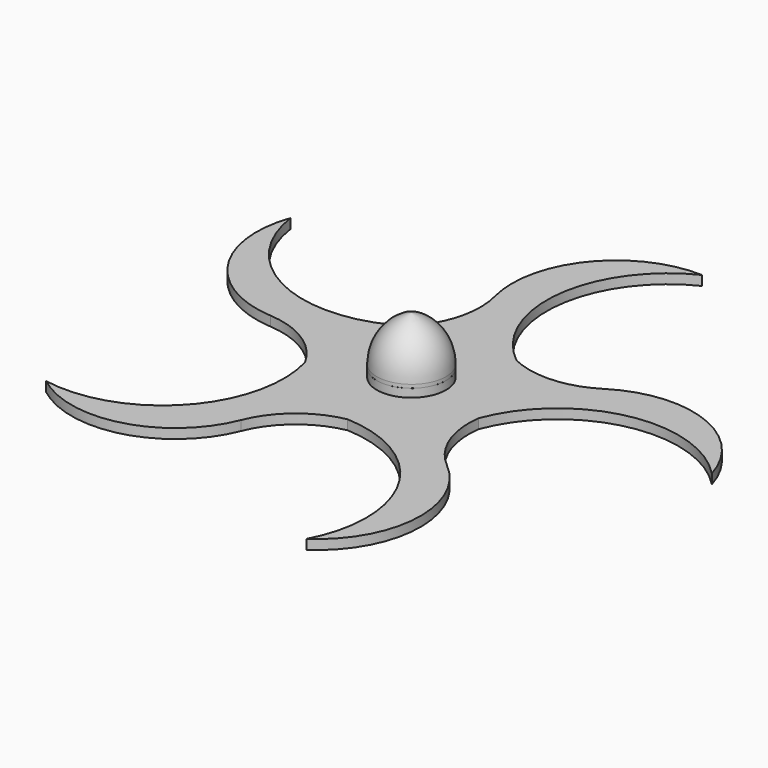
from build123d import *

# Parameters (mm, degrees)
F0_R     = 2.495
F1_DEPTH = 2.8
F3_DEPTH = 2.4
F5_DEPTH = 1
F6_W     = 7.505
F6_H     = 1


with BuildPart() as f1:
    # F0 (on Top) → F1 (new body)
    with BuildSketch(Plane.XY):
        with BuildLine():
            ThreePointArc((-22.7858082993, 10.2862500528), (-20.3407682899, 14.5345500576), (-17.1137876985, 18.2241123408))
            ThreePointArc((-17.1137876985, 18.2241123408), (-16.5666860585, 18.7537908739), (-16.0359703203, 19.2998864317))
            ThreePointArc((-16.0359703203, 19.2998864317), (-49.6996912533, 16.6900208036), (-69.9041814161, 43.7424898759))
            ThreePointArc((-69.9041814161, 43.7424898759), (-66.7598038962, 17.1440537541), (-43.6190942577, 3.6580806138))
            ThreePointArc((-43.6190942577, 3.6580806138), (-32.5771806136, 5.0068500705), (-22.7858082993, 10.2862500528))
        make_face()
        with BuildLine():
            ThreePointArc((-23.7810968086, -7.7109943963), (-24.9618581995, 1.3804474739), (-22.7858082993, 10.2862500528))
            ThreePointArc((-22.7858082993, 10.2862500528), (-32.5771806136, 5.0068500705), (-43.6190942577, 3.6580806138))
            ThreePointArc((-43.6190942577, 3.6580806138), (-31.8033376807, -0.2078903454), (-23.3106701049, -9.2871211714))
            ThreePointArc((-23.3106701049, -9.2871211714), (-23.5366233714, -8.4962939253), (-23.7810968086, -7.7109943963))
        make_face()
        with BuildLine():
            ThreePointArc((-14.6823545264, 20.2343387725), (-6.4007548293, 24.1667196288), (2.7416031459, 24.8492175368))
            ThreePointArc((2.7416031459, 24.8492175368), (-5.3051050528, 32.5299416652), (-10, 42.6146329052))
            ThreePointArc((-10, 42.6146329052), (-10.0254872889, 30.1825298915), (-16.0359703203, 19.2998864317))
            ThreePointArc((-16.0359703203, 19.2998864317), (-15.353672314, 19.7591598168), (-14.6823545264, 20.2343387725))
        make_face()
        with BuildLine():
            ThreePointArc((-17.1137876985, 18.2241123408), (-15.9298122297, 19.2676174533), (-14.6823545264, 20.2343387725))
            ThreePointArc((-14.6823545264, 20.2343387725), (-15.353672314, 19.7591598168), (-16.0359703203, 19.2998864317))
            ThreePointArc((-16.0359703203, 19.2998864317), (-16.5666860585, 18.7537908739), (-17.1137876985, 18.2241123408))
        make_face()
        with BuildLine():
            ThreePointArc((24.5572095563, -4.684384571), (24.8890562186, -2.3526326842), (25, 0))
            ThreePointArc((25, 0), (24.8697135657, 2.5489894392), (24.4802122271, 5.0714109788))
            ThreePointArc((24.4802122271, 5.0714109788), (21.0059741613, 13.5554066532), (14.7069026764, 20.2165034976))
            ThreePointArc((14.7069026764, 20.2165034976), (13.4020104362, 21.1041729586), (12.0437095584, 21.9077397299))
            ThreePointArc((12.0437095584, 21.9077397299), (7.5375354635, 23.8366432019), (2.7416031459, 24.8492175368))
            ThreePointArc((2.7416031459, 24.8492175368), (-6.4007548293, 24.1667196288), (-14.6823545264, 20.2343387725))
            ThreePointArc((-14.6823545264, 20.2343387725), (-15.9298122297, 19.2676174533), (-17.1137876985, 18.2241123408))
            ThreePointArc((-17.1137876985, 18.2241123408), (-20.3407682899, 14.5345500576), (-22.7858082993, 10.2862500528))
            ThreePointArc((-22.7858082993, 10.2862500528), (-24.9618581995, 1.3804474739), (-23.7810968086, -7.7109943963))
            ThreePointArc((-23.7810968086, -7.7109943963), (-23.2471758286, -9.1961304903), (-22.6206120324, -10.6446188885))
            ThreePointArc((-22.6206120324, -10.6446188885), (-20.1088216239, -14.8537972551), (-16.824007136, -18.4919653874))
            ThreePointArc((-16.824007136, -18.4919653874), (-9.0265219603, -23.3135561702), (-0.015171591, -24.9999953965))
            ThreePointArc((-0.015171591, -24.9999953965), (1.5622674252, -24.9511386612), (3.1334806162, -24.8028486112))
            ThreePointArc((3.1334806162, -24.8028486112), (7.9128330526, -23.7147016233), (12.3880000622, -21.714913181))
            ThreePointArc((12.3880000622, -21.714913181), (19.3831608278, -15.7890175857), (23.7717202497, -7.7398524773))
            ThreePointArc((23.7717202497, -7.7398524773), (24.2127101969, -6.2245212604), (24.5572095563, -4.684384571))
        make_face()
        Circle(F0_R, mode=Mode.SUBTRACT)
        with BuildLine():
            ThreePointArc((2.7416031459, 24.8492175368), (7.5375354635, 23.8366432019), (12.0437095584, 21.9077397299))
            ThreePointArc((12.0437095584, 21.9077397299), (12.7165274833, 21.5510948184), (13.3998954043, 21.2151069652))
            ThreePointArc((13.3998954043, 21.2151069652), (0.5151038299, 52.4247152891), (20, 80))
            ThreePointArc((20, 80), (-4.3249499065, 68.7901504845), (-10, 42.6146329052))
            ThreePointArc((-10, 42.6146329052), (-5.3051050528, 32.5299416652), (2.7416031459, 24.8492175368))
        make_face()
        with BuildLine():
            ThreePointArc((14.7069026764, 20.2165034976), (21.0059741613, 13.5554066532), (24.4802122271, 5.0714109788))
            ThreePointArc((24.4802122271, 5.0714109788), (29.2984453771, 15.0977595306), (37.4387543702, 22.6792109397))
            ThreePointArc((37.4387543702, 22.6792109397), (25.6072457824, 18.8617196848), (13.3998954043, 21.2151069652))
            ThreePointArc((13.3998954043, 21.2151069652), (14.0475320292, 20.7081262812), (14.7069026764, 20.2165034976))
        make_face()
        with BuildLine():
            ThreePointArc((24.4802122271, 5.0714109788), (24.8697135657, 2.5489894392), (25, 0))
            ThreePointArc((25, 0), (24.8890562186, -2.3526326842), (24.5572095563, -4.684384571))
            ThreePointArc((24.5572095563, -4.684384571), (24.4259322621, -5.4344817814), (24.3175611259, -6.1882292523))
            ThreePointArc((24.3175611259, -6.1882292523), (50.0180429279, 15.7102350956), (82.2648611911, 5.7002292241))
            ThreePointArc((82.2648611911, 5.7002292241), (64.0868378543, 25.3705973366), (37.4387543702, 22.6792109397))
            ThreePointArc((37.4387543702, 22.6792109397), (29.2984453771, 15.0977595306), (24.4802122271, 5.0714109788))
        make_face()
        with BuildLine():
            ThreePointArc((24.3175611259, -6.1882292523), (24.0355245661, -6.9608339317), (23.7717202497, -7.7398524773))
            ThreePointArc((23.7717202497, -7.7398524773), (19.3831608278, -15.7890175857), (12.3880000622, -21.714913181))
            ThreePointArc((12.3880000622, -21.714913181), (23.4125401133, -23.1990131213), (33.1384226973, -28.5981097064))
            ThreePointArc((33.1384226973, -28.5981097064), (25.8516355407, -18.52534604), (24.3175611259, -6.1882292523))
        make_face()
        with BuildLine():
            ThreePointArc((33.1384226973, -28.5981097064), (23.4125401133, -23.1990131213), (12.3880000622, -21.714913181))
            ThreePointArc((12.3880000622, -21.714913181), (7.9128330526, -23.7147016233), (3.1334806162, -24.8028486112))
            ThreePointArc((3.1334806162, -24.8028486112), (2.3795288615, -24.9097892705), (1.629183895, -25.0396429732))
            ThreePointArc((1.629183895, -25.0396429732), (30.3977467503, -42.7152560287), (30.8424802959, -76.4770645958))
            ThreePointArc((30.8424802959, -76.4770645958), (43.932793932, -53.1102590157), (33.1384226973, -28.5981097064))
        make_face()
        with BuildLine():
            ThreePointArc((1.629183895, -25.0396429732), (0.8072390901, -25.0101582411), (-0.015171591, -24.9999953965))
            ThreePointArc((-0.015171591, -24.9999953965), (-9.0265219603, -23.3135561702), (-16.824007136, -18.4919653874))
            ThreePointArc((-16.824007136, -18.4919653874), (-14.8286998241, -29.435538145), (-16.9580828098, -40.3538147522))
            ThreePointArc((-16.9580828098, -40.3538147522), (-9.6300563535, -30.3110131909), (1.629183895, -25.0396429732))
        make_face()
        with BuildLine():
            ThreePointArc((-16.9580828098, -40.3538147522), (-14.8286998241, -29.435538145), (-16.824007136, -18.4919653874))
            ThreePointArc((-16.824007136, -18.4919653874), (-20.1088216239, -14.8537972551), (-22.6206120324, -10.6446188885))
            ThreePointArc((-22.6206120324, -10.6446188885), (-22.9553025485, -9.9606146404), (-23.3106701049, -9.2871211714))
            ThreePointArc((-23.3106701049, -9.2871211714), (-31.2312022548, -42.1097151595), (-63.2031600709, -52.9656545041))
            ThreePointArc((-63.2031600709, -52.9656545041), (-36.9348779836, -58.1945425595), (-16.9580828098, -40.3538147522))
        make_face()
        with BuildLine():
            ThreePointArc((-23.3106701049, -9.2871211714), (-22.9553025485, -9.9606146404), (-22.6206120324, -10.6446188885))
            ThreePointArc((-22.6206120324, -10.6446188885), (-23.2471758286, -9.1961304903), (-23.7810968086, -7.7109943963))
            ThreePointArc((-23.7810968086, -7.7109943963), (-23.5366233714, -8.4962939253), (-23.3106701049, -9.2871211714))
        make_face()
        with BuildLine():
            ThreePointArc((1.629183895, -25.0396429732), (2.3795288615, -24.9097892705), (3.1334806162, -24.8028486112))
            ThreePointArc((3.1334806162, -24.8028486112), (1.5622674252, -24.9511386612), (-0.015171591, -24.9999953965))
            ThreePointArc((-0.015171591, -24.9999953965), (0.8072390901, -25.0101582411), (1.629183895, -25.0396429732))
        make_face()
        with BuildLine():
            ThreePointArc((24.3175611259, -6.1882292523), (24.4259322621, -5.4344817814), (24.5572095563, -4.684384571))
            ThreePointArc((24.5572095563, -4.684384571), (24.2127101969, -6.2245212604), (23.7717202497, -7.7398524773))
            ThreePointArc((23.7717202497, -7.7398524773), (24.0355245661, -6.9608339317), (24.3175611259, -6.1882292523))
        make_face()
        with BuildLine():
            ThreePointArc((12.0437095584, 21.9077397299), (13.4020104362, 21.1041729586), (14.7069026764, 20.2165034976))
            ThreePointArc((14.7069026764, 20.2165034976), (14.0475320292, 20.7081262812), (13.3998954043, 21.2151069652))
            ThreePointArc((13.3998954043, 21.2151069652), (12.7165274833, 21.5510948184), (12.0437095584, 21.9077397299))
        make_face()
    extrude(amount=F1_DEPTH)


with BuildPart() as f3:
    # F2 (on face) → F3 (new body)
    with BuildSketch(Plane.XY.offset(2.8)):
        with BuildLine():
            Line((10, 0), (2.55, 0))
            ThreePointArc((2.55, 0), (0, -2.55), (-2.55, 0))
            Line((-2.55, 0), (-10, 0))
            ThreePointArc((-10, 0), (0, -10), (10, 0))
        make_face()
        with BuildLine():
            ThreePointArc((-2.55, 0), (0, 2.55), (2.55, 0))
            Line((2.55, 0), (10, 0))
            ThreePointArc((10, 0), (0, 10), (-10, 0))
            Line((-10, 0), (-2.55, 0))
        make_face()
    extrude(amount=F3_DEPTH)


with BuildPart() as f5:
    # F4 (on face) → F5 (new body)
    with BuildSketch(Plane.XY.offset(5.2)):
        with BuildLine():
            ThreePointArc((10, 0), (0, 10), (-10, 0))
            Line((-10, 0), (-2.55, 0))
            ThreePointArc((-2.55, 0), (0, 2.55), (2.55, 0))
            Line((2.55, 0), (10, 0))
        make_face()
        with BuildLine():
            ThreePointArc((2.55, 0), (0, 2.55), (-2.55, 0))
            Line((-2.55, 0), (-2.495, 0))
            ThreePointArc((-2.495, 0), (0, 2.495), (2.495, 0))
            Line((2.495, 0), (2.55, 0))
        make_face()
    extrude(amount=F5_DEPTH)

    # F6 (on face) → F7 (revolve)
    with BuildSketch(Plane.XZ):
        with Locations((-6.2475, 5.7)):
            Rectangle(F6_W, F6_H)
        with BuildLine():
            ThreePointArc((0, 19.2180700541), (-7.2114289431, 14.4077729612), (-10, 6.2))
            Line((-10, 6.2), (-2.495, 6.2))
            Line((-2.495, 6.2), (-2.495, 13.6019121855))
            Line((-2.495, 13.6019121855), (0, 13.6019121855))
            Line((0, 13.6019121855), (0, 19.2180700541))
        make_face()
    revolve(axis=Axis((0, 0, 12.209035027), (0, 0, 1)))


solid = Compound([f1.part, f3.part, f5.part])
